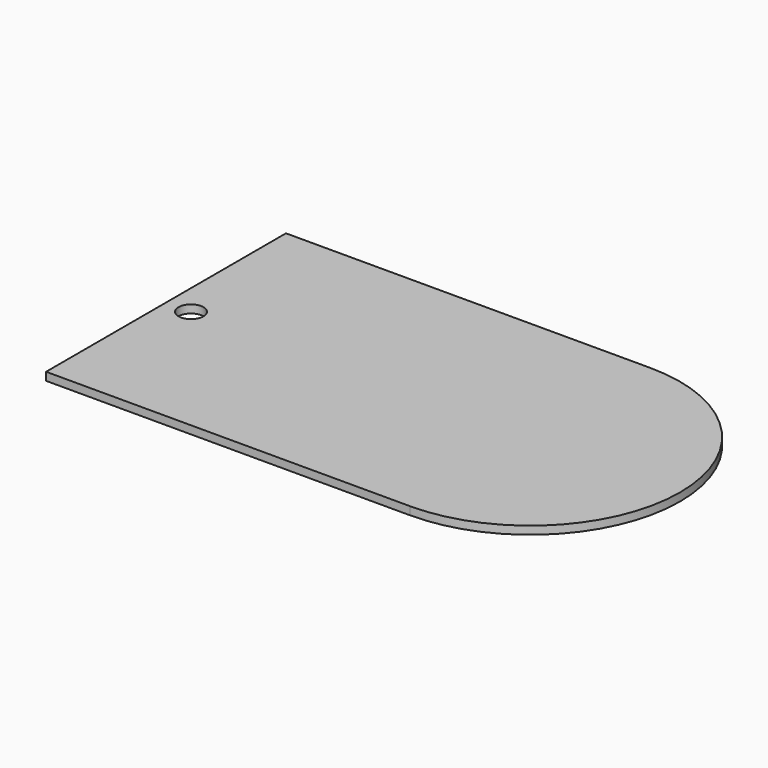
from build123d import *

# Parameters (mm, degrees)
F1_DEPTH = 28.575


# Not quite as in the source:
# - a feature names something its author has since deleted; it is built from what else it names


with BuildPart() as f1:
    # F0 (on Top) → F1 (new body)
    with BuildSketch(Plane.XY):
        with BuildLine():
            Line((304.8, 533.4), (-990.6, 533.4))
            Line((-990.6, 533.4), (-990.6, 0))
            Line((-990.6, 0), (-990.6, -533.4))
            Line((-990.6, -533.4), (304.8, -533.4))
            ThreePointArc((304.8, -533.4), (681.9707570849, -377.1707570849), (838.2, 0))
            ThreePointArc((838.2, 0), (681.9707570849, 377.1707570849), (304.8, 533.4))
        make_face()
        with BuildLine():
            ThreePointArc((-857.25, 0), (-901.7, -44.45), (-946.15, 0))
            ThreePointArc((-946.15, 0), (-901.7, 44.45), (-857.25, 0))
        make_face(mode=Mode.SUBTRACT)
    extrude(amount=F1_DEPTH)


solid = f1.part
